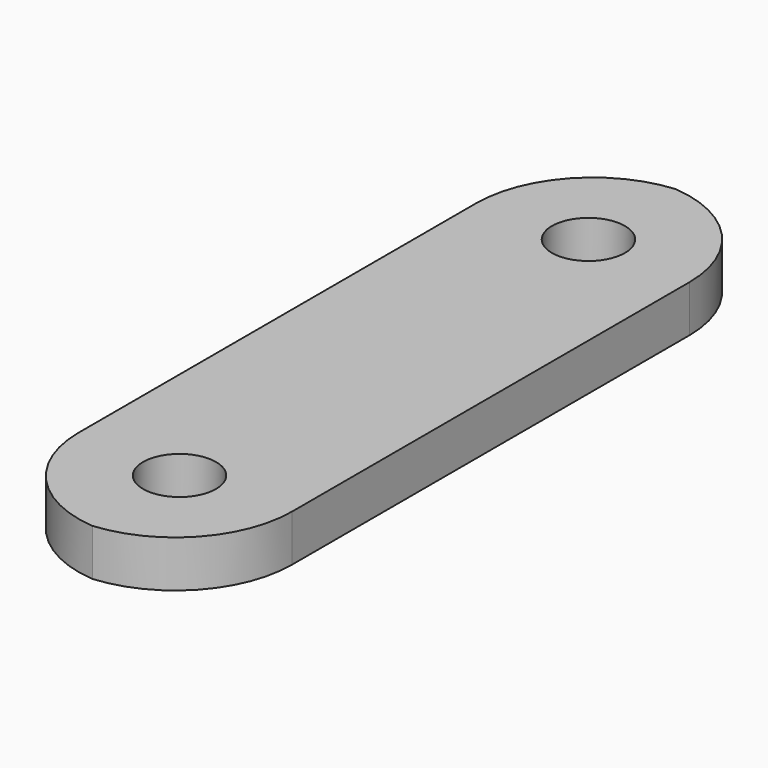
from build123d import *

# Parameters (mm, degrees)
F0_W        = 14.6192193359
F0_H        = 50
F0_R        = 2.5
F1_DEPTH    = 3.2
F2_T1_DEPTH = 43.2
F3_T1_DEPTH = 43.2


# Not quite as in the source:
# - a fillet or chamfer that OpenCascade refuses, or shapes differently, is made with other operations: its cross-section is extruded or revolved along the edge and cut away or added


with BuildPart() as f1:
    # F0 (on Top) → F1 (new body)
    with BuildSketch(Plane.XY):
        Rectangle(F0_W, F0_H)
        with Locations((0, -17.5)):
            Circle(F0_R, mode=Mode.SUBTRACT)
        with Locations((0, 17.5)):
            Circle(F0_R, mode=Mode.SUBTRACT)
    extrude(amount=F1_DEPTH)

    # F2: fillet of radius 8 on 2 edges, made by hand

    # F2_s2 → F2_t1 (cut)
    with BuildSketch(Plane.XY.offset(-20)):
        with BuildLine():
            ThreePointArc((-0.6903903321, -25), (4.9664639174, -22.6568542495), (7.3096096679, -17))
            Line((7.3096096679, -17), (7.3096096679, -25))
            Line((7.3096096679, -25), (-0.6903903321, -25))
        make_face()
        with BuildLine():
            ThreePointArc((0.6903903321, -25), (-4.9664639174, -22.6568542495), (-7.3096096679, -17))
            Line((-7.3096096679, -17), (-7.3096096679, -25))
            Line((-7.3096096679, -25), (0.6903903321, -25))
        make_face()
    extrude(amount=F2_T1_DEPTH, mode=Mode.SUBTRACT)

    # F3: fillet of radius 8 on 2 edges, made by hand

    # F3_s2 → F3_t1 (cut)
    with BuildSketch(Plane.XY.offset(-20)):
        with BuildLine():
            ThreePointArc((-0.6903903321, 25), (4.9664639174, 22.6568542495), (7.3096096679, 17))
            Line((7.3096096679, 17), (7.3096096679, 25))
            Line((7.3096096679, 25), (-0.6903903321, 25))
        make_face()
        with BuildLine():
            ThreePointArc((-7.3096096679, 17), (-4.9664639174, 22.6568542495), (0.6903903321, 25))
            Line((0.6903903321, 25), (-7.3096096679, 25))
            Line((-7.3096096679, 25), (-7.3096096679, 17))
        make_face()
    extrude(amount=F3_T1_DEPTH, mode=Mode.SUBTRACT)


solid = f1.part
